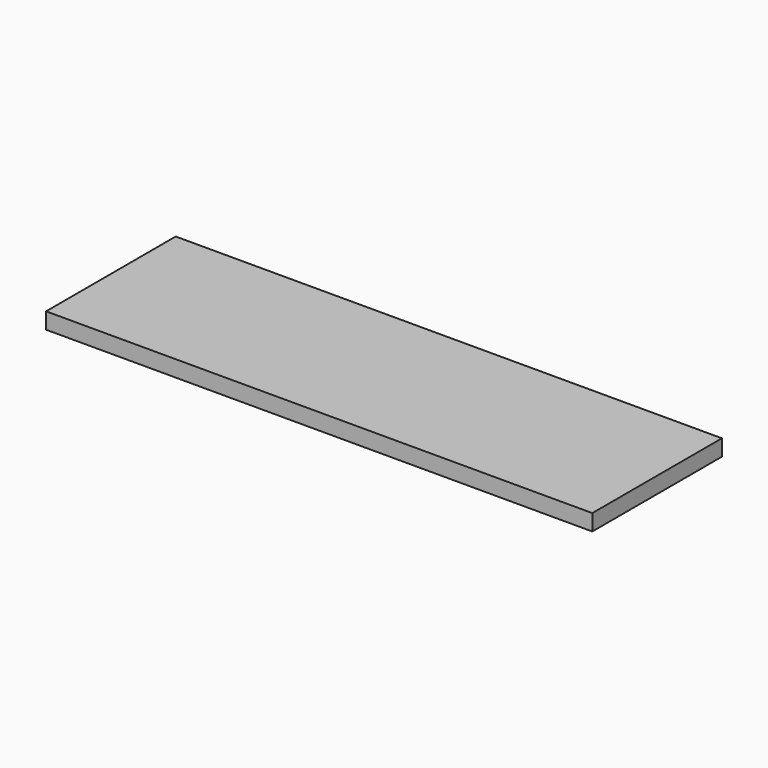
from build123d import *

# Parameters (mm, degrees)
F1_E0_BOTTOM_W = 85.6337100267
F1_E0_BOTTOM_H = 25.4
F2_DEPTH       = 2.54


with BuildPart() as f2:
    # F1_E0_bottom (on explicit) → F2 (new body)
    with BuildSketch(Plane(origin=(-42.8168550134, 0, -1.551660127), x_dir=(1, 0, 0), z_dir=(0, 0, -1))):
        with Locations((42.8168550134, 12.7)):
            Rectangle(F1_E0_BOTTOM_W, F1_E0_BOTTOM_H)
    extrude(amount=F2_DEPTH)


solid = f2.part
